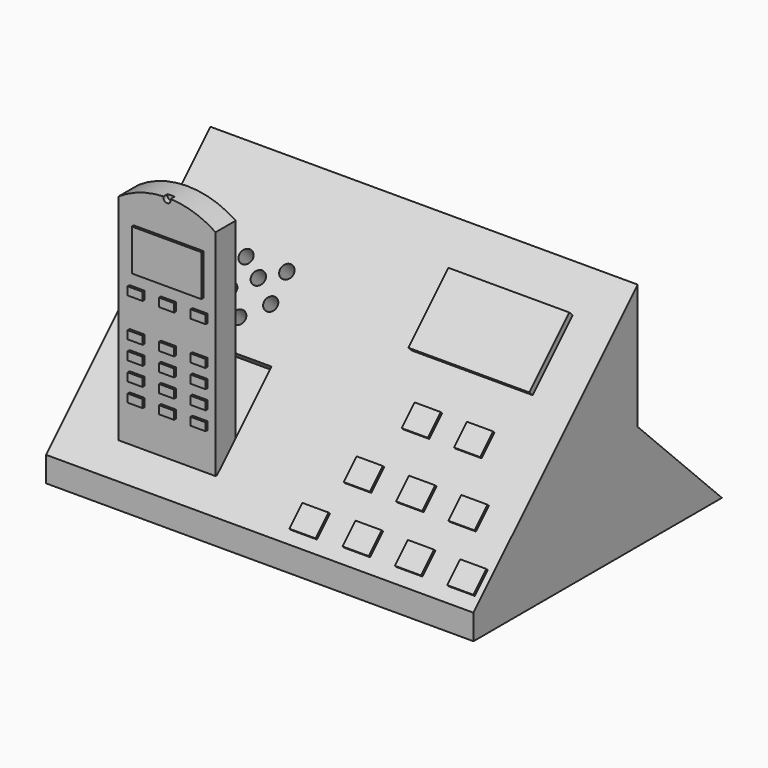
from build123d import *

# Parameters (mm, degrees)
F0_W        = 43.18
F0_H        = 20.7474600966
F1_DEPTH    = 25.4
F0_H_2      = 10.629949436
F2_DEPTH    = 12.7
F3_T1_DEPTH = 160.7573462098
F4_T4_DEPTH = 108.5007478943
F5_W        = 9.8024089821
F5_H        = 9.7506272141
F6_DEPTH    = 1.27
F7_W        = 2.6456220075
F7_H        = 2.3024471011
F7_W_2      = 2.6416
F7_H_2      = 2.3024467519
F7_H_3      = 2.3114
F8_DEPTH    = 0.254
F7_W_3      = 12.2105642222
F7_H_4      = 7.1489069227
F9_DEPTH    = 0.5842
F11_DEPTH   = 2.54
F13_W       = 1.524
F13_H       = 0.8168006316
F13_H_2     = 0.8128
F13_H_3     = 0.8049504831
F13_H_4     = 0.82042
F13_H_5     = 0.7896171883
F13_W_2     = 1.5263203532
F13_H_6     = 0.8140373975
F13_H_7     = 0.8394755423
F13_W_3     = 7.0272386074
F13_H_8     = 4.1753165424
F14_DEPTH   = 0.254
F15_DEPTH   = 0.508
F16_R       = 0.6775746303
F16_R_2     = 0.6719535835
F16_R_3     = 0.6676399197
F16_R_4     = 0.6773005459
F16_R_5     = 0.6826296901
F16_R_6     = 0.6703978175
F17_DEPTH   = 5.08


# Not quite as in the source:
# - a fillet or chamfer that OpenCascade refuses, or shapes differently, is made with other operations: its cross-section is extruded or revolved along the edge and cut away or added
# - a feature names something its author has since deleted; it is built from what else it names


with BuildPart() as f1:
    # F0 (on Top) → F1 (new body)
    with BuildSketch(Plane.XY):
        with Locations((0.5560219288, -5.7501500921)):
            Rectangle(F0_W, F0_H)
    extrude(amount=F1_DEPTH)

    # F0 (on Top) → F2 (join)
    with BuildSketch(Plane.XY):
        with Locations((0.5560219288, 9.9385546742)):
            Rectangle(F0_W, F0_H_2)
    extrude(amount=F2_DEPTH)

    # F3: chamfer of 22.86 on 1 edges, made by hand

    # F3_s2 → F3_t1 (cut)
    with BuildSketch(Plane.YZ.offset(-79.8226511761)):
        Polygon((-16.1238801405, 2.54), (6.7361198595, 25.4), (-16.1238801405, 25.4), align=None)
    extrude(amount=F3_T1_DEPTH, mode=Mode.SUBTRACT)

    # F4: chamfer of 12.7 on 1 edges, made by hand


with BuildPart() as f4_tool2:
    # F4_s3 → F4_t4 (new body)
    with BuildSketch(Plane.YZ.offset(54.806395876)):
        Polygon((2.5535293922, 12.7), (15.2535293922, 0), (15.2535293922, 12.7), align=None)
    extrude(amount=-F4_T4_DEPTH)

    split(bisect_by=Plane.XZ.offset(-4.6235799562), keep=Keep.BOTTOM)


with BuildPart() as f1_1:
    add(f1.part)

    # F4_t1: cut F4_tool2
    add(f4_tool2.part, mode=Mode.SUBTRACT)

    # F5 (on face) → F6 (cut)
    with BuildSketch(Plane(origin=(0, -9.3319400702, 9.3319400702), x_dir=(1, 0, 0), z_dir=(0, -0.7071067812, 0.7071067812))):
        with Locations((-10.4905848857, -1.5347840963)):
            Rectangle(F5_W, F5_H)
    extrude(amount=-F6_DEPTH, mode=Mode.SUBTRACT)

    # F7 (on face) → F8 (join)
    with BuildSketch(Plane(origin=(0, -9.3319400702, 9.3319400702), x_dir=(1, 0, 0), z_dir=(0, -0.7071067812, 0.7071067812))):
        with Locations((9.6429114781, 3.4242669353)):
            Rectangle(F7_W, F7_H)
        with Locations((14.9321444894, 3.4242669353)):
            Rectangle(F7_W_2, F7_H)
        with Locations((7.0073444894, -2.2598968935)):
            Rectangle(F7_W_2, F7_H_2)
        with Locations((12.2905444894, -2.2598968935)):
            Rectangle(F7_W_2, F7_H_2)
        with Locations((17.5737444894, -2.2598968935)):
            Rectangle(F7_W_2, F7_H_2)
        with Locations((4.3657444894, -7.2920206692)):
            Rectangle(F7_W_2, F7_H_3)
        with Locations((9.6489444894, -7.1481164303)):
            Rectangle(F7_W_2, F7_H_3)
        with Locations((14.9321444894, -7.1481164303)):
            Rectangle(F7_W_2, F7_H_3)
        with Locations((20.2153444894, -7.1481164303)):
            Rectangle(F7_W_2, F7_H_3)
    extrude(amount=F8_DEPTH)

    # F7 (on face) → F9 (join)
    with BuildSketch(Plane(origin=(0, -9.3319400702, 9.3319400702), x_dir=(1, 0, 0), z_dir=(0, -0.7071067812, 0.7071067812))):
        with Locations((11.7918266005, 12.0353225427)):
            Rectangle(F7_W_3, F7_H_4)
    extrude(amount=F9_DEPTH)

    # F16 (on face) → F17 (cut)
    with BuildSketch(Plane(origin=(0, -9.3319400702, 9.3319400702), x_dir=(1, 0, 0), z_dir=(0, -0.7071067812, 0.7071067812))):
        with Locations((-10.4905848857, 9.6622304991)):
            Circle(F16_R)
        with Locations((-8.3198184147, 8.0361571163)):
            Circle(F16_R_2)
        with Locations((-12.4481311068, 8.0361571163)):
            Circle(F16_R_3)
        with Locations((-10.4905848857, 6.1483839527)):
            Circle(F16_R_4)
        with Locations((-8.3198184147, 10.9258340672)):
            Circle(F16_R_5)
        with Locations((-12.4481311068, 10.9258340672)):
            Circle(F16_R_6)
    extrude(amount=-F17_DEPTH, mode=Mode.SUBTRACT)


with BuildPart() as f11:
    # F10 (on Front) → F11 (new body)
    with BuildSketch(Plane.XZ):
        with BuildLine():
            ThreePointArc((49.9308869097, 22.6276024803), (45.0286869097, 24.1148820906), (40.1264869097, 22.6276024803))
            Line((40.1264869097, 22.6276024803), (40.1264869097, 0.6058024803))
            ThreePointArc((40.1264869097, 0.6058024803), (45.0286869097, -0.2623128577), (49.9308869097, 0.6058024803))
            Line((49.9308869097, 0.6058024803), (49.9308869097, 22.6276024803))
        make_face()
    extrude(amount=F11_DEPTH)


with BuildPart() as f11_1:
    # F12: moved
    add(f11.part.moved(Location((-55.6006, -11.3792, 3.81))))

    # F13 (on face) → F14 (join)
    with BuildSketch(Plane.XZ.offset(13.9192)):
        with Locations((-13.5976772105, 14.5986099907)):
            Rectangle(F13_W, F13_H)
        with Locations((-10.4226772105, 14.596609675)):
            Rectangle(F13_W, F13_H_2)
        with Locations((-13.5976772105, 12.7249955591)):
            Rectangle(F13_W, F13_H_2)
        with Locations((-10.4226772105, 12.7209344334)):
            Rectangle(F13_W, F13_H_3)
        with Locations((-7.2476772105, 12.717009675)):
            Rectangle(F13_W, F13_H_2)
        with Locations((-7.2476772105, 14.596609675)):
            Rectangle(F13_W, F13_H_2)
        with Locations((-10.4226772105, 10.8414491918)):
            Rectangle(F13_W, F13_H_4)
        with Locations((-7.2476772105, 10.837409675)):
            Rectangle(F13_W, F13_H_2)
        with Locations((-7.2476772105, 8.9694010808)):
            Rectangle(F13_W, F13_H_5)
        with Locations((-10.4226772105, 8.9580391918)):
            Rectangle(F13_W, F13_H_2)
        with Locations((-13.5976772105, 8.9657955591)):
            Rectangle(F13_W, F13_H_2)
        with Locations((-13.5976772105, 10.8453955591)):
            Rectangle(F13_W, F13_H_2)
        with Locations((-13.5965170339, 18.4998149052)):
            Rectangle(F13_W_2, F13_H_6)
        with Locations((-10.4166828096, 18.5125339776)):
            Rectangle(F13_W_2, F13_H_7)
        with Locations((-7.240522633, 18.5125339776)):
            Rectangle(F13_W, F13_H_7)
        with Locations((-10.4216868058, 22.2753062844)):
            Rectangle(F13_W_3, F13_H_8)
    extrude(amount=F14_DEPTH)

    # F13 (on face) → F15 (cut)
    with BuildSketch(Plane.XZ.offset(13.9192)):
        with BuildLine():
            ThreePointArc((-10.9229198271, 27.9178969903), (-10.5719130903, 27.9248820906), (-10.2209063536, 27.9178969903))
            ThreePointArc((-10.2209063536, 27.9178969903), (-10.5719130903, 28.171962803), (-10.9229198271, 27.9178969903))
        make_face()
        with BuildLine():
            ThreePointArc((-10.9229198271, 27.9178969903), (-10.6303667733, 27.4376135857), (-10.2024120456, 27.8024617583))
            ThreePointArc((-10.2024120456, 27.8024617583), (-10.2070649178, 27.8609154413), (-10.2209063536, 27.9178969903))
            ThreePointArc((-10.2209063536, 27.9178969903), (-10.5719130903, 27.9248820906), (-10.9229198271, 27.9178969903))
        make_face()
    extrude(amount=-F15_DEPTH, mode=Mode.SUBTRACT)


solid = Compound([f1_1.part, f11_1.part])
